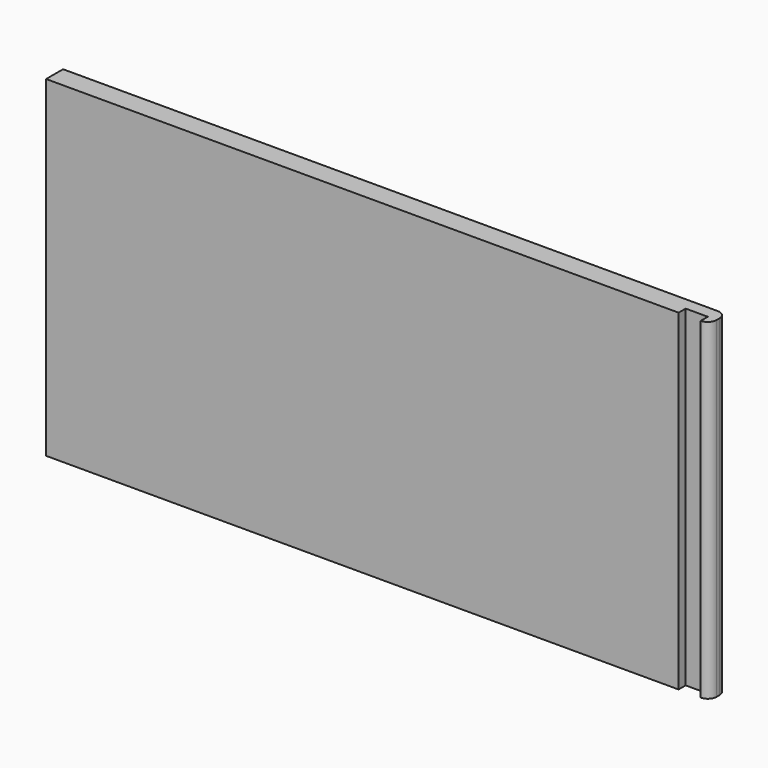
from build123d import *

# Parameters (mm, degrees)
F0_W     = 150
F0_H     = 75
F1_DEPTH = 4.8
F2_W     = 5
F2_H     = 75
F3_DEPTH = 2
F4_R     = 1.99999


# Not quite as in the source:
# - a fillet or chamfer is up to 0.001 mm smaller than in the source, because OpenCascade refuses the exact size


with BuildPart() as f1:
    # F0 (on Front) → F1 (new body)
    with BuildSketch(Plane.XZ):
        Rectangle(F0_W, F0_H)
    extrude(amount=F1_DEPTH)

    # F2 (on face) → F3 (cut)
    with BuildSketch(Plane.XZ.offset(4.8)):
        with Locations((70.5, 0)):
            Rectangle(F2_W, F2_H)
    extrude(amount=-F3_DEPTH, mode=Mode.SUBTRACT)

    # F4 (radius 2 in the source; OpenCascade refuses exactly that, so slightly less here)
    f4_edges = [f1.edges().sort_by_distance(p)[0] for p in [
        (75, 0, 0),
        (75, -4.8, 0),
    ]]
    fillet(f4_edges, radius=F4_R)


solid = f1.part
